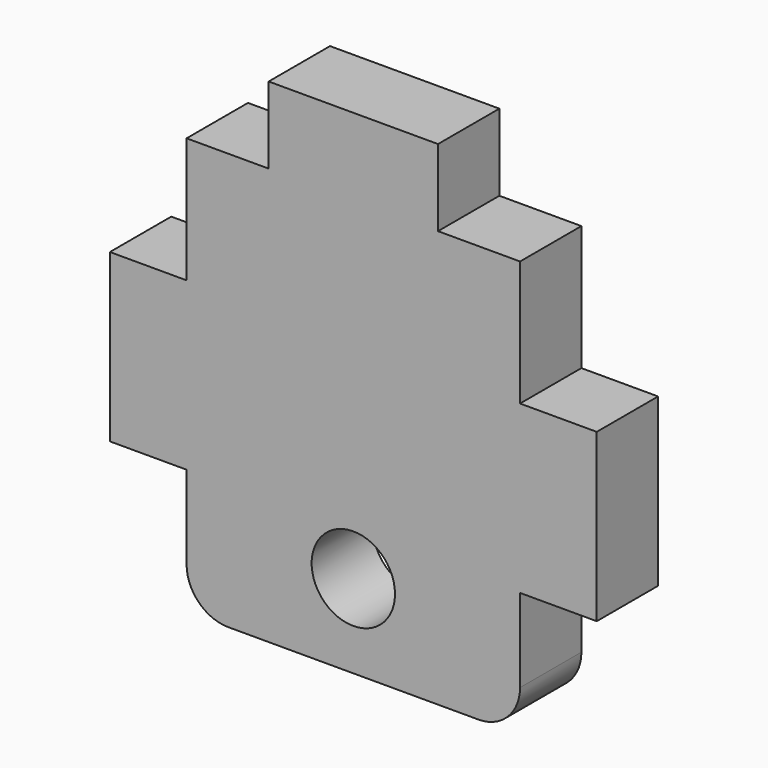
from build123d import *

# Parameters (mm, degrees)
F0_R     = 3.175
F1_DEPTH = 5.842
F2_R     = 3.175


with BuildPart() as f1:
    # F0 (on Front) → F1 (new body)
    with BuildSketch(Plane.XZ):
        Polygon((-12.7, 3.175), (-12.7, -6.35), (12.7, -6.35), (12.7, 3.175), (18.542, 3.175), (18.542, 15.875), (12.7, 15.875), (12.7, 25.4), (6.45, 25.4), (6.45, 31.242), (-6.45, 31.242), (-6.45, 25.4), (-12.7, 25.4), (-12.7, 15.875), (-18.542, 15.875), (-18.542, 3.175), align=None)
        Circle(F0_R, mode=Mode.SUBTRACT)
    extrude(amount=F1_DEPTH)

    # F2
    f2_edges = [f1.edges().sort_by_distance(p)[0] for p in [
        (-12.7, -2.921, -6.35),
        (12.7, -2.921, -6.35),
    ]]
    fillet(f2_edges, radius=F2_R)


solid = f1.part
